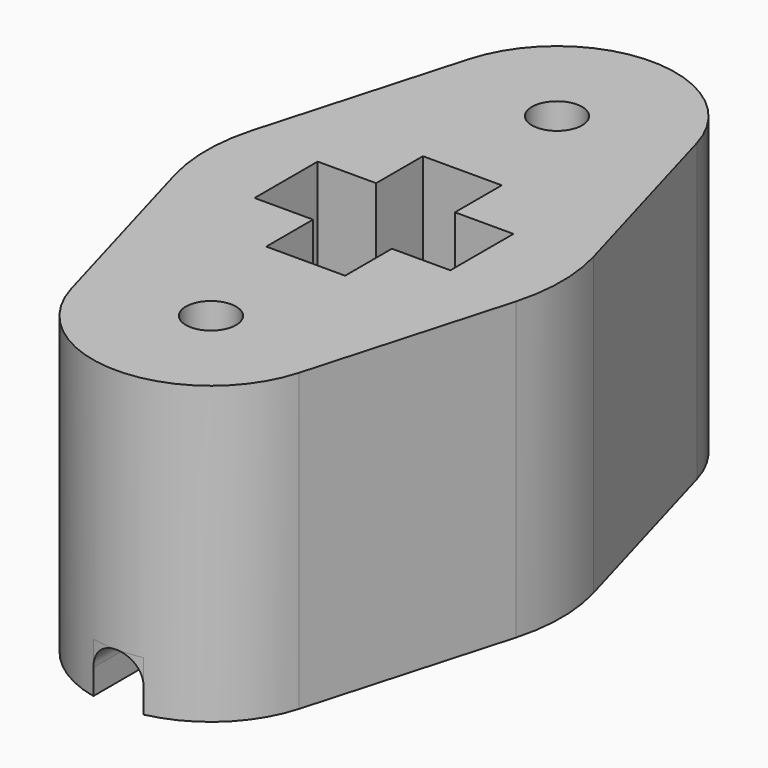
from build123d import *

# Parameters (mm, degrees)
F0_R         = 0.6731
F1_DEPTH     = 7.9375
F3_DEPTH     = 1.3462
F4_T4_DEPTH  = 6.4683311894
F4_S5_R      = 3.175
F4_T6_DEPTH  = 5
F4_S7_R      = 0.6731
F4_T8_DEPTH  = 5
F4_T12_DEPTH = 6.4683311894
F4_S13_R     = 3.175
F4_T14_DEPTH = 5
F4_S15_R     = 0.6731
F4_T16_DEPTH = 5
F4_T20_DEPTH = 6.4683311894
F4_S21_R     = 3.175
F4_T22_DEPTH = 5
F4_S23_R     = 0.6731
F4_T24_DEPTH = 5
F4_T28_DEPTH = 6.4683311894
F4_S29_R     = 3.175
F4_T30_DEPTH = 5
F4_S31_R     = 0.6731
F4_T32_DEPTH = 5


# Not quite as in the source:
# - a fillet or chamfer that OpenCascade refuses, or shapes differently, is made with other operations: its cross-section is extruded or revolved along the edge and cut away or added


with BuildPart() as f1:
    # F0 (on Top) → F1 (new body)
    with BuildSketch(Plane.XY):
        with BuildLine():
            ThreePointArc((-4.5806904159, 1.3033347856), (-4.7625, 0), (-4.5806904159, -1.3033347856))
            Line((-4.5806904159, -1.3033347856), (-3.0537936106, -6.6697545571))
            ThreePointArc((-3.0537936106, -6.6697545571), (0, -8.9758647), (3.0537936106, -6.6697545571))
            Line((3.0537936106, -6.6697545571), (4.5806904159, -1.3033347856))
            ThreePointArc((4.5806904159, -1.3033347856), (4.7625, 0), (4.5806904159, 1.3033347856))
            Line((4.5806904159, 1.3033347856), (3.0537936106, 6.6697545571))
            ThreePointArc((3.0537936106, 6.6697545571), (0, 8.9758647), (-3.0537936106, 6.6697545571))
            Line((-3.0537936106, 6.6697545571), (-4.5806904159, 1.3033347856))
        make_face()
        with Locations((0, -5.8008647)):
            Circle(F0_R, mode=Mode.SUBTRACT)
        Polygon((-1.0574147, 2.6258647), (1.0574147, 2.6258647), (1.0574147, 1.0574147), (2.6258647, 1.0574147), (2.6258647, -1.0574147), (1.0574147, -1.0574147), (1.0574147, -2.6258647), (-1.0574147, -2.6258647), (-1.0574147, -1.0574147), (-2.6258647, -1.0574147), (-2.6258647, 1.0574147), (-1.0574147, 1.0574147), align=None, mode=Mode.SUBTRACT)
        with Locations((0, 5.8008647)):
            Circle(F0_R, mode=Mode.SUBTRACT)
    extrude(amount=F1_DEPTH)

    # F2 (on face) → F3 (cut)
    with BuildSketch(Plane(origin=(0, 0, 0), x_dir=(1, 0, 0), z_dir=(0, 0, -1))):
        with BuildLine():
            Line((-0.6731, 5.8008647), (0.6731, 5.8008647))
            Line((0.6731, 5.8008647), (0.6731, 8.9036958894))
            ThreePointArc((0.6731, 8.9036958894), (0, 8.9758647), (-0.6731, 8.9036958894))
            Line((-0.6731, 8.9036958894), (-0.6731, 5.8008647))
        make_face()
        with BuildLine():
            Line((0.6731, -8.9036958894), (0.6731, -5.8008647))
            Line((0.6731, -5.8008647), (-0.6731, -5.8008647))
            Line((-0.6731, -5.8008647), (-0.6731, -8.9036958894))
            ThreePointArc((-0.6731, -8.9036958894), (0, -8.9758647), (0.6731, -8.9036958894))
        make_face()
    extrude(amount=-F3_DEPTH, mode=Mode.SUBTRACT)

    # F4: fillet of radius 0.6731 on 4 edges, made by hand


with BuildPart() as f4_tool2:
    # F4_s3 → F4_t4 (new body)
    with BuildSketch(Plane.XZ.offset(-10.5864458894)):
        with BuildLine():
            ThreePointArc((0.6731, 0.6731), (0.4759535744, 1.1490535744), (0, 1.3462))
            Line((0, 1.3462), (0.6731, 1.3462))
            Line((0.6731, 1.3462), (0.6731, 0.6731))
        make_face()
    extrude(amount=F4_T4_DEPTH)

    # F4_s5 → F4_t6 (intersect, symmetric)
    with BuildSketch(Plane.XY.offset(1)):
        with Locations((0, 5.8008647)):
            Circle(F4_S5_R)
    extrude(amount=F4_T6_DEPTH, both=True, mode=Mode.INTERSECT)

    # F4_s7 → F4_t8 (cut, symmetric)
    with BuildSketch(Plane.XY.offset(1)):
        with Locations((0, 5.8008647)):
            Circle(F4_S7_R)
    extrude(amount=F4_T8_DEPTH, both=True, mode=Mode.SUBTRACT)


with BuildPart() as f1_1:
    add(f1.part)

    # F4_t1: union F4_tool2
    add(f4_tool2.part)


with BuildPart() as f4_tool10:
    # F4_s11 → F4_t12 (new body)
    with BuildSketch(Plane.XZ.offset(-4.1181147)):
        with BuildLine():
            ThreePointArc((-0.6731, 0.6731), (-0.4759535744, 1.1490535744), (0, 1.3462))
            Line((0, 1.3462), (-0.6731, 1.3462))
            Line((-0.6731, 1.3462), (-0.6731, 0.6731))
        make_face()
    extrude(amount=-F4_T12_DEPTH)

    # F4_s13 → F4_t14 (intersect, symmetric)
    with BuildSketch(Plane.XY.offset(1)):
        with Locations((0, 5.8008647)):
            Circle(F4_S13_R)
    extrude(amount=F4_T14_DEPTH, both=True, mode=Mode.INTERSECT)

    # F4_s15 → F4_t16 (cut, symmetric)
    with BuildSketch(Plane.XY.offset(1)):
        with Locations((0, 5.8008647)):
            Circle(F4_S15_R)
    extrude(amount=F4_T16_DEPTH, both=True, mode=Mode.SUBTRACT)


with BuildPart() as f1_2:
    add(f1_1.part)

    # F4_t9: union F4_tool10
    add(f4_tool10.part)


with BuildPart() as f4_tool18:
    # F4_s19 → F4_t20 (new body)
    with BuildSketch(Plane.XZ.offset(4.1181147)):
        with BuildLine():
            ThreePointArc((0.6731, 0.6731), (0.4759535744, 1.1490535744), (0, 1.3462))
            Line((0, 1.3462), (0.6731, 1.3462))
            Line((0.6731, 1.3462), (0.6731, 0.6731))
        make_face()
    extrude(amount=F4_T20_DEPTH)

    # F4_s21 → F4_t22 (intersect, symmetric)
    with BuildSketch(Plane.XY.offset(1)):
        with Locations((0, -5.8008647)):
            Circle(F4_S21_R)
    extrude(amount=F4_T22_DEPTH, both=True, mode=Mode.INTERSECT)

    # F4_s23 → F4_t24 (cut, symmetric)
    with BuildSketch(Plane.XY.offset(1)):
        with Locations((0, -5.8008647)):
            Circle(F4_S23_R)
    extrude(amount=F4_T24_DEPTH, both=True, mode=Mode.SUBTRACT)


with BuildPart() as f1_3:
    add(f1_2.part)

    # F4_t17: union F4_tool18
    add(f4_tool18.part)


with BuildPart() as f4_tool26:
    # F4_s27 → F4_t28 (new body)
    with BuildSketch(Plane.XZ.offset(10.5864458894)):
        with BuildLine():
            ThreePointArc((-0.6731, 0.6731), (-0.4759535744, 1.1490535744), (0, 1.3462))
            Line((0, 1.3462), (-0.6731, 1.3462))
            Line((-0.6731, 1.3462), (-0.6731, 0.6731))
        make_face()
    extrude(amount=-F4_T28_DEPTH)

    # F4_s29 → F4_t30 (intersect, symmetric)
    with BuildSketch(Plane.XY.offset(1)):
        with Locations((0, -5.8008647)):
            Circle(F4_S29_R)
    extrude(amount=F4_T30_DEPTH, both=True, mode=Mode.INTERSECT)

    # F4_s31 → F4_t32 (cut, symmetric)
    with BuildSketch(Plane.XY.offset(1)):
        with Locations((0, -5.8008647)):
            Circle(F4_S31_R)
    extrude(amount=F4_T32_DEPTH, both=True, mode=Mode.SUBTRACT)


with BuildPart() as f1_4:
    add(f1_3.part)

    # F4_t25: union F4_tool26
    add(f4_tool26.part)


solid = f1_4.part
